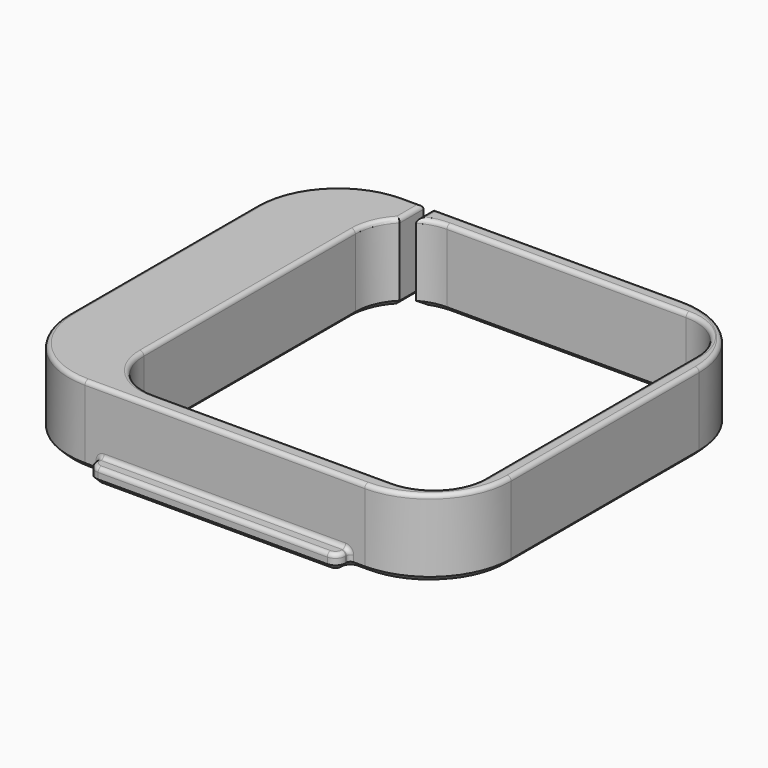
from build123d import *

# Parameters (mm, degrees)
F1_DEPTH     = 7.62
F3_DEPTH     = 1.5
F4_F1_R      = 0.4
F4_F2_R      = 0.4
F5_T1_DEPTH  = 1.0466503546
F5_T3_DEPTH  = 0.1
F5_T5_DEPTH  = 3.285841494
F5_T7_DEPTH  = 5.5009687737
F5_T9_DEPTH  = 18.2066992909
F5_T11_DEPTH = 26
F5_T13_DEPTH = 23.5
F5_T15_DEPTH = 1.0466503546
F5_T17_DEPTH = 1.0844961911
F5_T19_DEPTH = 0.1
F5_T21_DEPTH = 4.741555969
F5_T23_DEPTH = 22.5310076177
F5_T25_DEPTH = 25.785841494
F5_T27_DEPTH = 23.1
F5_T29_DEPTH = 1.0844961911
F5_T32_ANGLE = 90
F5_T34_ANGLE = 90
F5_T36_ANGLE = 90
F5_T38_ANGLE = 60.3091715098
F5_T40_ANGLE = 90
F5_T42_ANGLE = 90
F5_T44_ANGLE = 90
F5_T46_ANGLE = 90
F5_T48_ANGLE = 90
F5_T50_ANGLE = 90
F5_T52_ANGLE = 90
F5_T54_ANGLE = 44.7353156515
F5_T56_ANGLE = 90
F5_T58_ANGLE = 90
F5_T60_ANGLE = 90
F5_T62_ANGLE = 90
F5_T64_ANGLE = 90


# Not quite as in the source:
# - a fillet or chamfer that OpenCascade refuses, or shapes differently, is made with other operations: its cross-section is extruded or revolved along the edge and cut away or added


with BuildPart() as f1:
    # F0 (on Top) → F1 (new body)
    with BuildSketch(Plane.XY):
        with BuildLine():
            Line((-13.1889366657, 21.7579442412), (-14.6889366657, 21.7579442412))
            ThreePointArc((-14.6889366657, 21.7579442412), (-20.3457909151, 19.4147984907), (-22.6889366657, 13.7579442412))
            Line((-22.6889366657, 13.7579442412), (-22.6889366657, -9.3420557588))
            ThreePointArc((-22.6889366657, -9.3420557588), (-20.3457909151, -14.9989100083), (-14.6889366657, -17.3420557588))
            Line((-14.6889366657, -17.3420557588), (12.8110633343, -17.3420557588))
            ThreePointArc((12.8110633343, -17.3420557588), (18.4679175838, -14.9989100083), (20.8110633343, -9.3420557588))
            Line((20.8110633343, -9.3420557588), (20.8110633343, 13.7579442412))
            ThreePointArc((20.8110633343, 13.7579442412), (18.4679175838, 19.4147984907), (12.8110633343, 21.7579442412))
            Line((12.8110633343, 21.7579442412), (-11.6889366657, 21.7579442412))
            Line((-11.6889366657, 21.7579442412), (-11.6889366657, 19.5880712601))
            ThreePointArc((-11.6889366657, 19.5880712601), (-10.4830318912, 20.0875733726), (-9.1889366657, 20.2579442412))
            Line((-9.1889366657, 20.2579442412), (14.3110633343, 20.2579442412))
            ThreePointArc((14.3110633343, 20.2579442412), (17.8465972403, 18.7934781471), (19.3110633343, 15.2579442412))
            Line((19.3110633343, 15.2579442412), (19.3110633343, -10.7420557588))
            ThreePointArc((19.3110633343, -10.7420557588), (17.8465972403, -14.2775896648), (14.3110633343, -15.7420557588))
            Line((14.3110633343, -15.7420557588), (-9.1889366657, -15.7420557588))
            ThreePointArc((-9.1889366657, -15.7420557588), (-12.7244705716, -14.2775896648), (-14.1889366657, -10.7420557588))
            Line((-14.1889366657, -10.7420557588), (-14.1889366657, 15.2579442412))
            ThreePointArc((-14.1889366657, 15.2579442412), (-13.7987088943, 17.1944359143), (-12.6889366657, 18.8286584554))
            Line((-12.6889366657, 18.8286584554), (-12.6889366657, 21.7579442412))
            Line((-12.6889366657, 21.7579442412), (-13.1889366657, 21.7579442412))
        make_face()
    extrude(amount=F1_DEPTH)

    # F2 (on Top) → F3 (join)
    with BuildSketch(Plane.XY):
        with BuildLine():
            Line((-22.6889366657, -7.8954054043), (-22.6889366657, 12.3112938866))
            Line((-22.6889366657, 12.3112938866), (-23.1889366657, 12.3112938866))
            ThreePointArc((-23.1889366657, 12.3112938866), (-23.8960434468, 12.0184006678), (-24.1889366657, 11.3112938866))
            Line((-24.1889366657, 11.3112938866), (-24.1889366657, -6.8954054043))
            ThreePointArc((-24.1889366657, -6.8954054043), (-23.8960434468, -7.6025121855), (-23.1889366657, -7.8954054043))
            Line((-23.1889366657, -7.8954054043), (-22.6889366657, -7.8954054043))
        make_face()
        with BuildLine():
            Line((11.3265671432, -17.3420557588), (-13.2044404745, -17.3420557588))
            Line((-13.2044404745, -17.3420557588), (-13.2044404745, -17.8420557588))
            ThreePointArc((-13.2044404745, -17.8420557588), (-12.9115472557, -18.54916254), (-12.2044404745, -18.8420557588))
            Line((-12.2044404745, -18.8420557588), (10.3265671432, -18.8420557588))
            ThreePointArc((10.3265671432, -18.8420557588), (11.0336739244, -18.54916254), (11.3265671432, -17.8420557588))
            Line((11.3265671432, -17.8420557588), (11.3265671432, -17.3420557588))
        make_face()
    extrude(amount=F3_DEPTH)

    # F4: fillet of radius 0.4 on 32 edges, made by hand

    # F4_f1
    f4_f1_edges = [f1.edges().sort_by_distance(p)[0] for p in [
        (-12.6889366657, 20.2933013483, 7.62),
        (-13.6889366657, 21.7579442412, 7.62),
        (-20.3457909151, 19.4147984907, 7.62),
        (-22.6889366657, 2.2079442412, 7.62),
        (-20.3457909151, -14.9989100083, 7.62),
        (-0.9389366657, -17.3420557588, 7.62),
        (18.4679175838, -14.9989100083, 7.62),
        (20.8110633343, 2.2079442412, 7.62),
        (18.4679175838, 19.4147984907, 7.62),
        (0.5610633343, 21.7579442412, 7.62),
        (-11.6889366657, 20.6730077506, 7.62),
        (-10.4830318912, 20.0875733726, 7.62),
        (2.5610633343, 20.2579442412, 7.62),
        (17.8465972403, 18.7934781471, 7.62),
        (19.3110633343, 2.2579442412, 7.62),
        (17.8465972403, -14.2775896648, 7.62),
        (2.5610633343, -15.7420557588, 7.62),
        (-12.7244705716, -14.2775896648, 7.62),
        (-14.1889366657, 2.2579442412, 7.62),
        (-13.7987088943, 17.1944359143, 7.62),
        (11.0336739244, -18.54916254, 1.5),
        (11.3265671432, -17.5920557588, 1.5),
        (-13.2044404745, -17.5920557588, 1.5),
        (-12.9115472557, -18.54916254, 1.5),
        (-0.9389366657, -18.8420557588, 1.5),
        (-22.9389366657, 12.3112938866, 1.5),
        (-23.8960434468, 12.0184006678, 1.5),
        (-24.1889366657, 2.2079442412, 1.5),
        (-23.8960434468, -7.6025121855, 1.5),
        (-22.9389366657, -7.8954054043, 1.5),
    ]]
    fillet(f4_f1_edges, radius=F4_F1_R)

    # F4_f2
    f4_f2_edges = [f1.edges().sort_by_distance(p)[0] for p in [
        (-0.9389366657, -17.3420557588, 1.5),
        (-22.6889366657, 2.2079442412, 1.5),
        (-22.6889366657, -7.7782481167, 1.3828427125),
        (-22.6889366657, 12.1941365991, 1.3828427125),
        (11.2094098557, -17.3420557588, 1.3828427125),
        (-13.087283187, -17.3420557588, 1.3828427125),
    ]]
    fillet(f4_f2_edges, radius=F4_F2_R)

    # F5: chamfer of 0.5 on 36 edges, made by hand

    # F5_s2 → F5_t1 (cut)
    with BuildSketch(Plane.XZ.offset(-13.7579442412)):
        Polygon((-22.1889366657, 0), (-22.6889366657, 0.5), (-22.6889366657, 0), align=None)
    extrude(amount=F5_T1_DEPTH, mode=Mode.SUBTRACT)

    # F5_s4 → F5_t3 (cut)
    with BuildSketch(Plane.YZ.offset(-23.1889366657)):
        Polygon((11.8112938866, 0), (12.3112938866, 0.5), (12.3112938866, 0), align=None)
        Polygon((-7.3954054043, 0), (-7.8954054043, 0.5), (-7.8954054043, 0), align=None)
    extrude(amount=F5_T3_DEPTH, mode=Mode.SUBTRACT)

    # F5_s6 → F5_t5 (cut)
    with BuildSketch(Plane.YZ.offset(-14.6889366657)):
        Polygon((21.2579442412, 0), (21.7579442412, 0.5), (21.7579442412, 0), align=None)
    extrude(amount=F5_T5_DEPTH, mode=Mode.SUBTRACT)

    # F5_s8 → F5_t7 (cut)
    with BuildSketch(Plane.XZ.offset(-23.0437857351)):
        Polygon((-13.1889366657, 0), (-12.6889366657, 0.5), (-12.6889366657, 0), align=None)
    extrude(amount=F5_T7_DEPTH, mode=Mode.SUBTRACT)

    # F5_s10 → F5_t9 (cut)
    with BuildSketch(Plane.XZ.offset(-11.3112938866)):
        Polygon((-23.6889366657, 0), (-24.1889366657, 0.5), (-24.1889366657, 0), align=None)
    extrude(amount=F5_T9_DEPTH, mode=Mode.SUBTRACT)

    # F5_s12 → F5_t11 (cut)
    with BuildSketch(Plane.XZ.offset(-15.2579442412)):
        Polygon((-14.6889366657, 0), (-14.1889366657, 0.5), (-14.1889366657, 0), align=None)
        Polygon((19.8110633343, 0), (19.3110633343, 0.5), (19.3110633343, 0), align=None)
    extrude(amount=F5_T11_DEPTH, mode=Mode.SUBTRACT)

    # F5_s14 → F5_t13 (cut)
    with BuildSketch(Plane.YZ.offset(-9.1889366657)):
        Polygon((-16.2420557588, 0), (-15.7420557588, 0.5), (-15.7420557588, 0), align=None)
        Polygon((20.7579442412, 0), (20.2579442412, 0.5), (20.2579442412, 0), align=None)
    extrude(amount=F5_T13_DEPTH, mode=Mode.SUBTRACT)

    # F5_s16 → F5_t15 (cut)
    with BuildSketch(Plane.XZ.offset(8.2954054043)):
        Polygon((-22.1889366657, 0), (-22.6889366657, 0.5), (-22.6889366657, 0), align=None)
    extrude(amount=F5_T15_DEPTH, mode=Mode.SUBTRACT)

    # F5_s18 → F5_t17 (cut)
    with BuildSketch(Plane.YZ.offset(-14.6889366657)):
        Polygon((-16.8420557588, 0), (-17.3420557588, 0.5), (-17.3420557588, 0), align=None)
    extrude(amount=F5_T17_DEPTH, mode=Mode.SUBTRACT)

    # F5_s20 → F5_t19 (cut)
    with BuildSketch(Plane.XZ.offset(17.7420557588)):
        Polygon((-12.7044404745, 0), (-13.2044404745, 0.5), (-13.2044404745, 0), align=None)
        Polygon((10.8265671432, 0), (11.3265671432, 0.5), (11.3265671432, 0), align=None)
    extrude(amount=F5_T19_DEPTH, mode=Mode.SUBTRACT)

    # F5_s22 → F5_t21 (cut)
    with BuildSketch(Plane.XZ.offset(-23.0437857351)):
        Polygon((-11.1889366657, 0), (-11.6889366657, 0.5), (-11.6889366657, 0), align=None)
    extrude(amount=F5_T21_DEPTH, mode=Mode.SUBTRACT)

    # F5_s24 → F5_t23 (cut)
    with BuildSketch(Plane.YZ.offset(-12.2044404745)):
        Polygon((-18.3420557588, 0), (-18.8420557588, 0.5), (-18.8420557588, 0), align=None)
    extrude(amount=F5_T23_DEPTH, mode=Mode.SUBTRACT)

    # F5_s26 → F5_t25 (cut)
    with BuildSketch(Plane.YZ.offset(-12.9747781596)):
        Polygon((21.2579442412, 0), (21.7579442412, 0.5), (21.7579442412, 0), align=None)
    extrude(amount=F5_T25_DEPTH, mode=Mode.SUBTRACT)

    # F5_s28 → F5_t27 (cut)
    with BuildSketch(Plane.XZ.offset(-13.7579442412)):
        Polygon((20.3110633343, 0), (20.8110633343, 0.5), (20.8110633343, 0), align=None)
    extrude(amount=F5_T27_DEPTH, mode=Mode.SUBTRACT)

    # F5_s30 → F5_t29 (cut)
    with BuildSketch(Plane.YZ.offset(11.7265671432)):
        Polygon((-16.8420557588, 0), (-17.3420557588, 0.5), (-17.3420557588, 0), align=None)
    extrude(amount=F5_T29_DEPTH, mode=Mode.SUBTRACT)

    # F5_s31 → F5_t32 (revolve, cut)
    with BuildSketch(Plane.XZ.offset(-12.7112938866)):
        Polygon((-22.1889366657, 0), (-22.6889366657, 0.5), (-22.6889366657, 0), align=None)
    revolve(axis=Axis((-23.0889366657, 12.7112938866, 0), (0, 0, -1)), revolution_arc=F5_T32_ANGLE, mode=Mode.SUBTRACT)

    # F5_s33 → F5_t34 (revolve, cut)
    with BuildSketch(Plane.YZ.offset(-14.6889366657)):
        Polygon((21.2579442412, 0), (21.7579442412, 0.5), (21.7579442412, 0), align=None)
    revolve(axis=Axis((-14.6889366657, 13.7579442412, 0), (0, 0, 1)), revolution_arc=F5_T34_ANGLE, mode=Mode.SUBTRACT)

    # F5_s35 → F5_t36 (revolve, cut)
    with BuildSketch(Plane.YZ.offset(-23.1889366657)):
        Polygon((11.8112938866, 0), (12.3112938866, 0.5), (12.3112938866, 0), align=None)
    revolve(axis=Axis((-23.1889366657, 11.3112938866, 0), (0, 0, 1)), revolution_arc=F5_T36_ANGLE, mode=Mode.SUBTRACT)

    # F5_s37 → F5_t38 (revolve, cut)
    with BuildSketch(Plane.XZ.offset(-15.2579442412)):
        Polygon((-14.6889366657, 0), (-14.1889366657, 0.5), (-14.1889366657, 0), align=None)
    revolve(axis=Axis((-9.1889366657, 15.2579442412, 0), (0, 0, -1)), revolution_arc=F5_T38_ANGLE, mode=Mode.SUBTRACT)

    # F5_s39 → F5_t40 (revolve, cut)
    with BuildSketch(Plane.XZ.offset(6.8954054043)):
        Polygon((-23.6889366657, 0), (-24.1889366657, 0.5), (-24.1889366657, 0), align=None)
    revolve(axis=Axis((-23.1889366657, -6.8954054043, 0), (0, 0, 1)), revolution_arc=F5_T40_ANGLE, mode=Mode.SUBTRACT)

    # F5_s41 → F5_t42 (revolve, cut)
    with BuildSketch(Plane.YZ.offset(-9.1889366657)):
        Polygon((-16.2420557588, 0), (-15.7420557588, 0.5), (-15.7420557588, 0), align=None)
    revolve(axis=Axis((-9.1889366657, -10.7420557588, 0), (0, 0, -1)), revolution_arc=F5_T42_ANGLE, mode=Mode.SUBTRACT)

    # F5_s43 → F5_t44 (revolve, cut)
    with BuildSketch(Plane.XZ.offset(8.2954054043)):
        Polygon((-22.1889366657, 0), (-22.6889366657, 0.5), (-22.6889366657, 0), align=None)
    revolve(axis=Axis((-23.0889366657, -8.2954054043, 0), (0, 0, 1)), revolution_arc=F5_T44_ANGLE, mode=Mode.SUBTRACT)

    # F5_s45 → F5_t46 (revolve, cut)
    with BuildSketch(Plane.XZ.offset(10.7420557588)):
        Polygon((19.8110633343, 0), (19.3110633343, 0.5), (19.3110633343, 0), align=None)
    revolve(axis=Axis((14.3110633343, -10.7420557588, 0), (0, 0, -1)), revolution_arc=F5_T46_ANGLE, mode=Mode.SUBTRACT)

    # F5_s47 → F5_t48 (revolve, cut)
    with BuildSketch(Plane.XZ.offset(9.3420557588)):
        Polygon((-22.1889366657, 0), (-22.6889366657, 0.5), (-22.6889366657, 0), align=None)
    revolve(axis=Axis((-14.6889366657, -9.3420557588, 0), (0, 0, 1)), revolution_arc=F5_T48_ANGLE, mode=Mode.SUBTRACT)

    # F5_s49 → F5_t50 (revolve, cut)
    with BuildSketch(Plane.YZ.offset(14.3110633343)):
        Polygon((20.7579442412, 0), (20.2579442412, 0.5), (20.2579442412, 0), align=None)
    revolve(axis=Axis((14.3110633343, 15.2579442412, 0), (0, 0, -1)), revolution_arc=F5_T50_ANGLE, mode=Mode.SUBTRACT)

    # F5_s51 → F5_t52 (revolve, cut)
    with BuildSketch(Plane.YZ.offset(-13.6044404745)):
        Polygon((-16.8420557588, 0), (-17.3420557588, 0.5), (-17.3420557588, 0), align=None)
    revolve(axis=Axis((-13.6044404745, -17.7420557588, 0), (0, 0, -1)), revolution_arc=F5_T52_ANGLE, mode=Mode.SUBTRACT)

    # F5_s53 → F5_t54 (revolve, cut)
    with BuildSketch(Plane(origin=(2.9917294423, 2.9642150856, 0), x_dir=(0, 0, 1), z_dir=(-0.7103657844, -0.7038326878, 0))):
        Polygon((0, 22.8061955202), (0.5, 22.3061955202), (0, 22.3061955202), align=None)
    revolve(axis=Axis((-9.1889366657, 15.2579442412, 0), (0, 0, -1)), revolution_arc=F5_T54_ANGLE, mode=Mode.SUBTRACT)

    # F5_s55 → F5_t56 (revolve, cut)
    with BuildSketch(Plane.XZ.offset(17.8420557588)):
        Polygon((-12.7044404745, 0), (-13.2044404745, 0.5), (-13.2044404745, 0), align=None)
    revolve(axis=Axis((-12.2044404745, -17.8420557588, 0), (0, 0, 1)), revolution_arc=F5_T56_ANGLE, mode=Mode.SUBTRACT)

    # F5_s57 → F5_t58 (revolve, cut)
    with BuildSketch(Plane.YZ.offset(10.3265671432)):
        Polygon((-18.3420557588, 0), (-18.8420557588, 0.5), (-18.8420557588, 0), align=None)
    revolve(axis=Axis((10.3265671432, -17.8420557588, 0), (0, 0, 1)), revolution_arc=F5_T58_ANGLE, mode=Mode.SUBTRACT)

    # F5_s59 → F5_t60 (revolve, cut)
    with BuildSketch(Plane.XZ.offset(-13.7579442412)):
        Polygon((20.3110633343, 0), (20.8110633343, 0.5), (20.8110633343, 0), align=None)
    revolve(axis=Axis((12.8110633343, 13.7579442412, 0), (0, 0, 1)), revolution_arc=F5_T60_ANGLE, mode=Mode.SUBTRACT)

    # F5_s61 → F5_t62 (revolve, cut)
    with BuildSketch(Plane.YZ.offset(11.7265671432)):
        Polygon((-16.8420557588, 0), (-17.3420557588, 0.5), (-17.3420557588, 0), align=None)
    revolve(axis=Axis((11.7265671432, -17.7420557588, 0), (0, 0, 1)), revolution_arc=F5_T62_ANGLE, mode=Mode.SUBTRACT)

    # F5_s63 → F5_t64 (revolve, cut)
    with BuildSketch(Plane.YZ.offset(12.8110633343)):
        Polygon((-16.8420557588, 0), (-17.3420557588, 0.5), (-17.3420557588, 0), align=None)
    revolve(axis=Axis((12.8110633343, -9.3420557588, 0), (0, 0, 1)), revolution_arc=F5_T64_ANGLE, mode=Mode.SUBTRACT)


solid = f1.part
